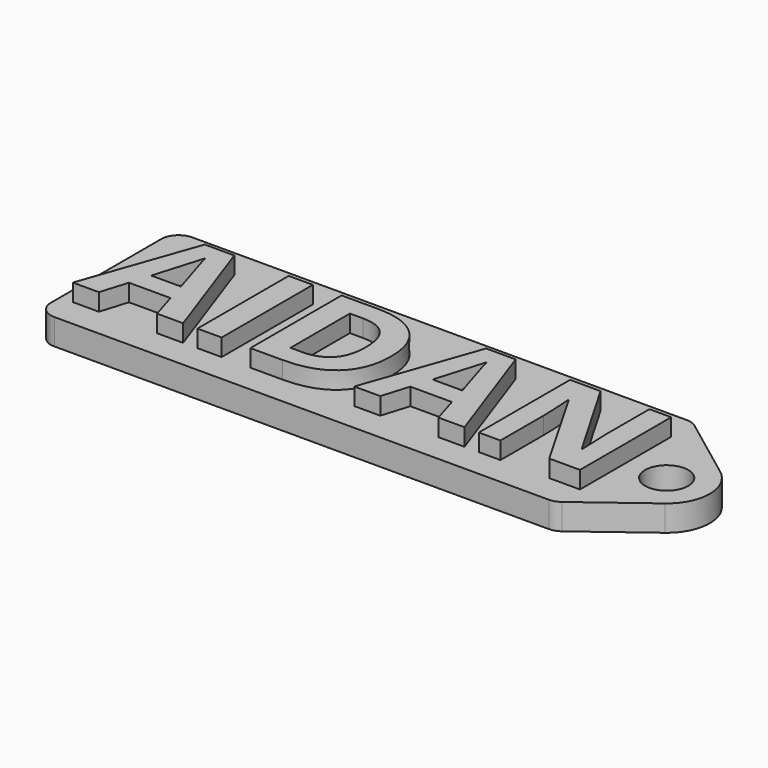
from build123d import *

# Parameters (mm, degrees)
F0_R         = 2.5
F1_DEPTH     = 3
F2_TEXT_SIZE = 18.5220914528
F3_DEPTH     = 2


# Not quite as in the source:
# - Text() gives the source's letters only with a copy of the font that has no kerning and outlines rounded to 1/6400 em; it was checked with that copy


with BuildPart() as f1:
    # F0 (on Top) → F1 (new body)
    with BuildSketch(Plane.XY):
        with BuildLine():
            Line((-28, -10), (29.3333333333, -10))
            ThreePointArc((29.3333333333, -10), (29.9657888654, -9.8973665961), (30.5333333333, -9.6))
            Line((30.5333333333, -9.6), (38, -4))
            ThreePointArc((38, -4), (39.472135955, -2.2360679775), (40, 0))
            ThreePointArc((40, 0), (39.472135955, 2.2360679775), (38, 4))
            Line((38, 4), (30.5333333333, 9.6))
            ThreePointArc((30.5333333333, 9.6), (29.9657888654, 9.8973665961), (29.3333333333, 10))
            Line((29.3333333333, 10), (-28, 10))
            ThreePointArc((-28, 10), (-29.4142135624, 9.4142135624), (-30, 8))
            Line((-30, 8), (-30, -8))
            ThreePointArc((-30, -8), (-29.4142135624, -9.4142135624), (-28, -10))
        make_face()
        with Locations((35, 0)):
            Circle(F0_R, mode=Mode.SUBTRACT)
    extrude(amount=F1_DEPTH)

    # F2 (on face) → F3 (join)
    with BuildSketch(Plane.XY.offset(3)):
        with Locations((-28.5173784941, -6.667952923)):
            Text('AIDAN', F2_TEXT_SIZE, font='Open Sans', font_style=FontStyle.BOLD, text_align=(TextAlign.LEFT, TextAlign.BOTTOM))
    extrude(amount=F3_DEPTH)


solid = f1.part
